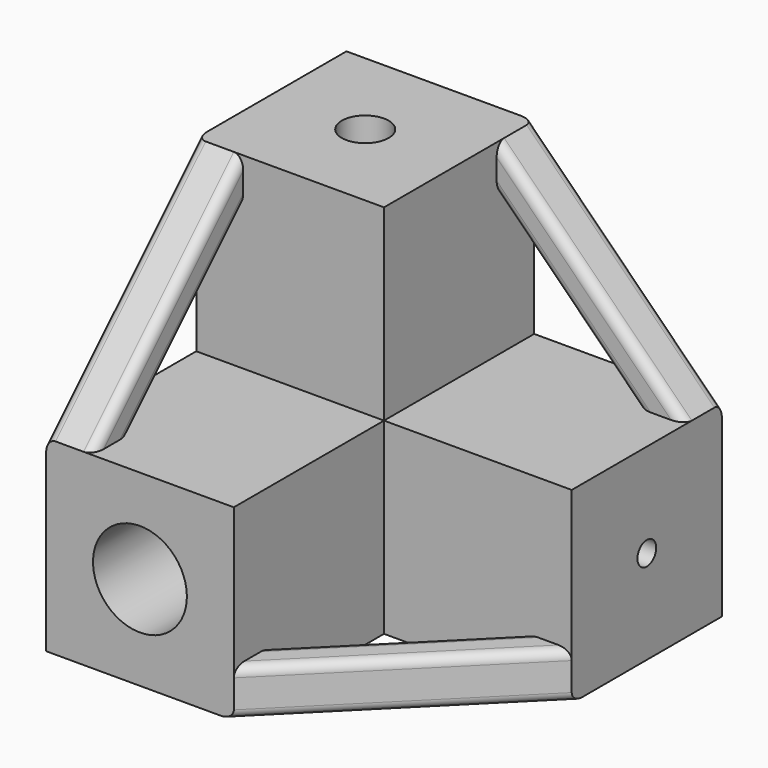
from build123d import *

# Parameters (mm, degrees)
F0_W          = 25.4
F0_H          = 25.4
F1_DEPTH      = 12.7
F2_R          = 3.175
F3_DEPTH      = 5.08
F4_R          = 1.5875
F5_DEPTH      = 5.08
F6_R          = 6.35
F7_DEPTH      = 12.7
F8_SIZE       = 1.27
F9_SIZE       = 0.396875
F10_SIZE      = 0.79375
F11_W         = 25.4
F11_H         = 25.4
F11_R         = 1.5875
F12_DEPTH     = 25.4
F13_W         = 25.4
F13_H         = 25.4
F13_R         = 6.35
F14_DEPTH     = 25.4
F15_W         = 25.4
F15_H         = 25.4
F15_R         = 3.175
F16_DEPTH     = 25.4
F18_DEPTH     = 6.35
F20_DEPTH     = 6.35
F22_DEPTH     = 6.35
F23_T1_DEPTH  = 42.2710244843
F23_T3_DEPTH  = 42.2710244843
F23_T5_DEPTH  = 42.2710244843
F23_T10_DEPTH = 42.2710244843
F23_T16_DEPTH = 33.2907683632
F23_T22_DEPTH = 33.2907683632
F23_T28_DEPTH = 42.2710244843
F23_T34_DEPTH = 33.2907683632
F23_T40_DEPTH = 33.2907683632
F23_T46_DEPTH = 42.2710244843
F23_T52_DEPTH = 33.2907683632
F23_T58_DEPTH = 33.2907683632


# Not quite as in the source:
# - a fillet or chamfer that OpenCascade refuses, or shapes differently, is made with other operations: its cross-section is extruded or revolved along the edge and cut away or added


with BuildPart() as f1:
    # F0 (on Top) → F1 (new body, symmetric)
    with BuildSketch(Plane.XY):
        Rectangle(F0_W, F0_H)
    extrude(amount=F1_DEPTH, both=True)

    # F2 (on face) → F3 (cut)
    with BuildSketch(Plane.XY.offset(12.7)):
        Circle(F2_R)
    extrude(amount=-F3_DEPTH, mode=Mode.SUBTRACT)

    # F4 (on face) → F5 (cut)
    with BuildSketch(Plane.YZ.offset(12.7)):
        Circle(F4_R)
    extrude(amount=-F5_DEPTH, mode=Mode.SUBTRACT)

    # F6 (on face) → F7 (cut)
    with BuildSketch(Plane.XZ.offset(12.7)):
        Circle(F6_R)
    extrude(amount=-F7_DEPTH, mode=Mode.SUBTRACT)

    # F8
    f8_edges = [f1.edges().sort_by_distance(p)[0] for p in [
        (-6.35, 0, 0),
    ]]
    chamfer(f8_edges, length=F8_SIZE)

    # F9
    f9_edges = [f1.edges().sort_by_distance(p)[0] for p in [
        (7.62, -1.5875, 0),
    ]]
    chamfer(f9_edges, length=F9_SIZE)

    # F10
    f10_edges = [f1.edges().sort_by_distance(p)[0] for p in [
        (-3.175, 0, 7.62),
    ]]
    chamfer(f10_edges, length=F10_SIZE)

    # F11 (on face) → F12 (join)
    with BuildSketch(Plane.YZ.offset(12.7)):
        Rectangle(F11_W, F11_H)
        Circle(F11_R, mode=Mode.SUBTRACT)
    extrude(amount=F12_DEPTH)

    # F13 (on face) → F14 (join)
    with BuildSketch(Plane.XZ.offset(12.7)):
        Rectangle(F13_W, F13_H)
        Circle(F13_R, mode=Mode.SUBTRACT)
    extrude(amount=F14_DEPTH)

    # F15 (on face) → F16 (join)
    with BuildSketch(Plane.XY.offset(12.7)):
        Rectangle(F15_W, F15_H)
        Circle(F15_R, mode=Mode.SUBTRACT)
    extrude(amount=F16_DEPTH)

    # F17 (on face) → F18 (join)
    with BuildSketch(Plane(origin=(0, 0, -12.7), x_dir=(1, 0, 0), z_dir=(0, 0, -1))):
        Polygon((38.1, 12.7), (12.7, 38.1), (12.7, 31.75), (31.75, 12.7), align=None)
    extrude(amount=-F18_DEPTH)

    # F19 (on face) → F20 (join)
    with BuildSketch(Plane(origin=(0, 12.7, 0), x_dir=(-1, 0, 0), z_dir=(0, 1, 0))):
        Polygon((-12.7, 38.1), (-38.1, 12.7), (-31.75, 12.7), (-12.7, 31.75), align=None)
    extrude(amount=-F20_DEPTH)

    # F21 (on face) → F22 (join)
    with BuildSketch(Plane(origin=(-12.7, 0, 0), x_dir=(0, -1, 0), z_dir=(-1, 0, 0))):
        Polygon((38.1, 12.7), (12.7, 38.1), (12.7, 31.75), (31.75, 12.7), align=None)
    extrude(amount=-F22_DEPTH)

    # F23: fillet of radius 1.27 on 12 edges, made by hand

    # F23_s2 → F23_t1 (cut)
    with BuildSketch(Plane(origin=(-14.9450640303, 0, 14.9450640303), x_dir=(0, 1, 0), z_dir=(0.7071067812, 0, -0.7071067812))):
        with BuildLine():
            ThreePointArc((11.43, 35.9210244843), (12.3280256121, 35.5490500964), (12.7, 34.6510244843))
            Line((12.7, 34.6510244843), (12.7, 35.9210244843))
            Line((12.7, 35.9210244843), (11.43, 35.9210244843))
        make_face()
    extrude(amount=F23_T1_DEPTH, mode=Mode.SUBTRACT)

    # F23_s4 → F23_t3 (cut)
    with BuildSketch(Plane(origin=(0, -14.9450640303, -14.9450640303), x_dir=(1, 0, 0), z_dir=(0, 0.7071067812, 0.7071067812))):
        with BuildLine():
            ThreePointArc((-11.43, -35.9210244843), (-12.3280256121, -35.5490500964), (-12.7, -34.6510244843))
            Line((-12.7, -34.6510244843), (-12.7, -35.9210244843))
            Line((-12.7, -35.9210244843), (-11.43, -35.9210244843))
        make_face()
    extrude(amount=F23_T3_DEPTH, mode=Mode.SUBTRACT)

    # F23_s6 → F23_t5 (cut)
    with BuildSketch(Plane(origin=(14.9450640303, 14.9450640303, 0), x_dir=(0, 0, 1), z_dir=(-0.7071067812, -0.7071067812, 0))):
        with BuildLine():
            ThreePointArc((-11.43, -35.9210244843), (-12.3280256121, -35.5490500964), (-12.7, -34.6510244843))
            Line((-12.7, -34.6510244843), (-12.7, -35.9210244843))
            Line((-12.7, -35.9210244843), (-11.43, -35.9210244843))
        make_face()
    extrude(amount=F23_T5_DEPTH, mode=Mode.SUBTRACT)


with BuildPart() as f23_tool8:
    # F23_s9 → F23_t10 (new body)
    with BuildSketch(Plane(origin=(-14.9450640303, 0, 14.9450640303), x_dir=(0, 1, 0), z_dir=(0.7071067812, 0, -0.7071067812))):
        with BuildLine():
            ThreePointArc((7.62, 35.9210244843), (6.7219743879, 35.5490500964), (6.35, 34.6510244843))
            Line((6.35, 34.6510244843), (6.35, 35.9210244843))
            Line((6.35, 35.9210244843), (7.62, 35.9210244843))
        make_face()
    extrude(amount=F23_T10_DEPTH)

    split(bisect_by=Plane.YZ.offset(12.7), keep=Keep.TOP)

    split(bisect_by=Plane.XY.offset(12.7), keep=Keep.TOP)


with BuildPart() as f1_1:
    add(f1.part)

    # F23_t7: cut F23_tool8
    add(f23_tool8.part, mode=Mode.SUBTRACT)


with BuildPart() as f23_tool14:
    # F23_s15 → F23_t16 (new body)
    with BuildSketch(Plane(origin=(11.7700640303, 0, -11.7700640303), x_dir=(0, 1, 0), z_dir=(-0.7071067812, 0, 0.7071067812))):
        with BuildLine():
            ThreePointArc((12.7, -32.7008964237), (12.3280256121, -31.8028708116), (11.43, -31.4308964237))
            Line((11.43, -31.4308964237), (12.7, -31.4308964237))
            Line((12.7, -31.4308964237), (12.7, -32.7008964237))
        make_face()
    extrude(amount=F23_T16_DEPTH)

    split(bisect_by=Plane.YZ.offset(12.7), keep=Keep.TOP)

    split(bisect_by=Plane.XY.offset(12.7), keep=Keep.TOP)


with BuildPart() as f1_2:
    add(f1_1.part)

    # F23_t13: cut F23_tool14
    add(f23_tool14.part, mode=Mode.SUBTRACT)


with BuildPart() as f23_tool20:
    # F23_s21 → F23_t22 (new body)
    with BuildSketch(Plane(origin=(11.7700640303, 0, -11.7700640303), x_dir=(0, 1, 0), z_dir=(-0.7071067812, 0, 0.7071067812))):
        with BuildLine():
            ThreePointArc((7.62, -31.4308964237), (6.7219743879, -31.8028708116), (6.35, -32.7008964237))
            Line((6.35, -32.7008964237), (6.35, -31.4308964237))
            Line((6.35, -31.4308964237), (7.62, -31.4308964237))
        make_face()
    extrude(amount=F23_T22_DEPTH)

    split(bisect_by=Plane.YZ.offset(12.7), keep=Keep.TOP)

    split(bisect_by=Plane.XY.offset(12.7), keep=Keep.TOP)


with BuildPart() as f1_3:
    add(f1_2.part)

    # F23_t19: cut F23_tool20
    add(f23_tool20.part, mode=Mode.SUBTRACT)


with BuildPart() as f23_tool26:
    # F23_s27 → F23_t28 (new body)
    with BuildSketch(Plane(origin=(0, -14.9450640303, -14.9450640303), x_dir=(1, 0, 0), z_dir=(0, 0.7071067812, 0.7071067812))):
        with BuildLine():
            ThreePointArc((-7.62, -35.9210244843), (-6.7219743879, -35.5490500964), (-6.35, -34.6510244843))
            Line((-6.35, -34.6510244843), (-6.35, -35.9210244843))
            Line((-6.35, -35.9210244843), (-7.62, -35.9210244843))
        make_face()
    extrude(amount=F23_T28_DEPTH)

    split(bisect_by=Plane.XZ.offset(12.7), keep=Keep.TOP)

    split(bisect_by=Plane.XY.offset(12.7), keep=Keep.TOP)


with BuildPart() as f1_4:
    add(f1_3.part)

    # F23_t25: cut F23_tool26
    add(f23_tool26.part, mode=Mode.SUBTRACT)


with BuildPart() as f23_tool32:
    # F23_s33 → F23_t34 (new body)
    with BuildSketch(Plane(origin=(0, 11.7700640303, 11.7700640303), x_dir=(1, 0, 0), z_dir=(0, -0.7071067812, -0.7071067812))):
        with BuildLine():
            ThreePointArc((-6.35, 32.7008964237), (-6.7219743879, 31.8028708116), (-7.62, 31.4308964237))
            Line((-7.62, 31.4308964237), (-6.35, 31.4308964237))
            Line((-6.35, 31.4308964237), (-6.35, 32.7008964237))
        make_face()
    extrude(amount=F23_T34_DEPTH)

    split(bisect_by=Plane.XZ.offset(12.7), keep=Keep.TOP)

    split(bisect_by=Plane.XY.offset(12.7), keep=Keep.TOP)


with BuildPart() as f1_5:
    add(f1_4.part)

    # F23_t31: cut F23_tool32
    add(f23_tool32.part, mode=Mode.SUBTRACT)


with BuildPart() as f23_tool38:
    # F23_s39 → F23_t40 (new body)
    with BuildSketch(Plane(origin=(0, 11.7700640303, 11.7700640303), x_dir=(1, 0, 0), z_dir=(0, -0.7071067812, -0.7071067812))):
        with BuildLine():
            ThreePointArc((-12.7, 32.7008964237), (-12.3280256121, 31.8028708116), (-11.43, 31.4308964237))
            Line((-11.43, 31.4308964237), (-12.7, 31.4308964237))
            Line((-12.7, 31.4308964237), (-12.7, 32.7008964237))
        make_face()
    extrude(amount=F23_T40_DEPTH)

    split(bisect_by=Plane.XZ.offset(12.7), keep=Keep.TOP)

    split(bisect_by=Plane.XY.offset(12.7), keep=Keep.TOP)


with BuildPart() as f1_6:
    add(f1_5.part)

    # F23_t37: cut F23_tool38
    add(f23_tool38.part, mode=Mode.SUBTRACT)


with BuildPart() as f23_tool44:
    # F23_s45 → F23_t46 (new body)
    with BuildSketch(Plane(origin=(14.9450640303, 14.9450640303, 0), x_dir=(0, 0, 1), z_dir=(-0.7071067812, -0.7071067812, 0))):
        with BuildLine():
            ThreePointArc((-7.62, -35.9210244843), (-6.7219743879, -35.5490500964), (-6.35, -34.6510244843))
            Line((-6.35, -34.6510244843), (-6.35, -35.9210244843))
            Line((-6.35, -35.9210244843), (-7.62, -35.9210244843))
        make_face()
    extrude(amount=F23_T46_DEPTH)

    split(bisect_by=Plane.YZ.offset(12.7), keep=Keep.TOP)

    split(bisect_by=Plane.XZ.offset(12.7), keep=Keep.TOP)


with BuildPart() as f1_7:
    add(f1_6.part)

    # F23_t43: cut F23_tool44
    add(f23_tool44.part, mode=Mode.SUBTRACT)


with BuildPart() as f23_tool50:
    # F23_s51 → F23_t52 (new body)
    with BuildSketch(Plane(origin=(-11.7700640303, -11.7700640303, 0), x_dir=(0, 0, 1), z_dir=(0.7071067812, 0.7071067812, 0))):
        with BuildLine():
            ThreePointArc((-12.7, 32.7008964237), (-12.3280256121, 31.8028708116), (-11.43, 31.4308964237))
            Line((-11.43, 31.4308964237), (-12.7, 31.4308964237))
            Line((-12.7, 31.4308964237), (-12.7, 32.7008964237))
        make_face()
    extrude(amount=F23_T52_DEPTH)

    split(bisect_by=Plane.YZ.offset(12.7), keep=Keep.TOP)

    split(bisect_by=Plane.XZ.offset(12.7), keep=Keep.TOP)


with BuildPart() as f1_8:
    add(f1_7.part)

    # F23_t49: cut F23_tool50
    add(f23_tool50.part, mode=Mode.SUBTRACT)


with BuildPart() as f23_tool56:
    # F23_s57 → F23_t58 (new body)
    with BuildSketch(Plane(origin=(-11.7700640303, -11.7700640303, 0), x_dir=(0, 0, 1), z_dir=(0.7071067812, 0.7071067812, 0))):
        with BuildLine():
            ThreePointArc((-6.35, 32.7008964237), (-6.7219743879, 31.8028708116), (-7.62, 31.4308964237))
            Line((-7.62, 31.4308964237), (-6.35, 31.4308964237))
            Line((-6.35, 31.4308964237), (-6.35, 32.7008964237))
        make_face()
    extrude(amount=F23_T58_DEPTH)

    split(bisect_by=Plane.YZ.offset(12.7), keep=Keep.TOP)

    split(bisect_by=Plane.XZ.offset(12.7), keep=Keep.TOP)


with BuildPart() as f1_9:
    add(f1_8.part)

    # F23_t55: cut F23_tool56
    add(f23_tool56.part, mode=Mode.SUBTRACT)


solid = f1_9.part
